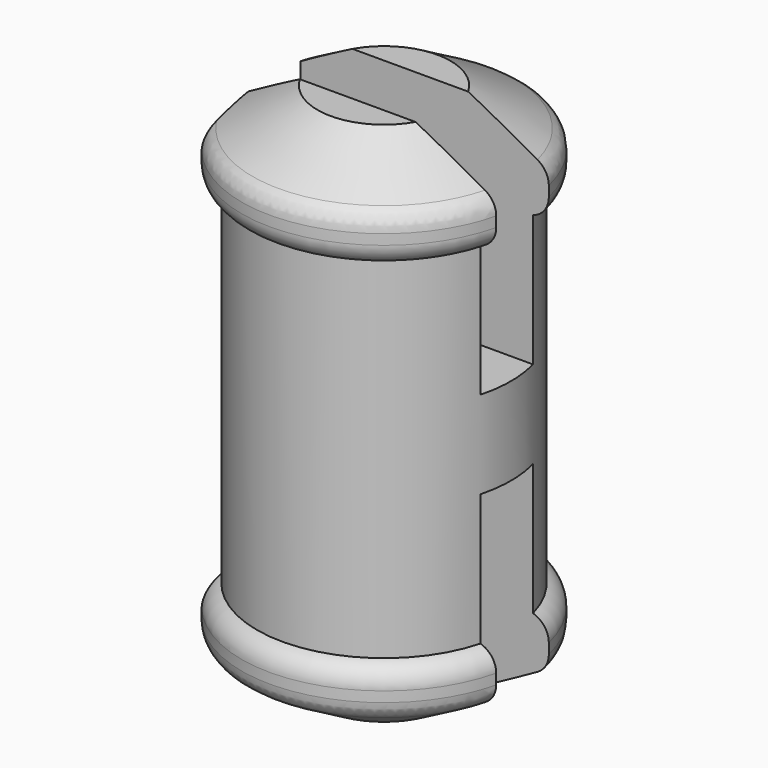
from build123d import *

# Parameters (mm, degrees)
F0_R         = 3.25
F1_DEPTH     = 2
F2_R         = 2.9
F3_DEPTH     = 8
F4_R         = 3.25
F5_DEPTH     = 2
F8_DEPTH     = 5
F10_DEPTH    = 5
F11_C1_SIZE2 = 1
F11_C1_SIZE  = 1.7320508076
F11_C2_SIZE2 = 1
F11_C2_SIZE  = 1.7320508076
F12_C1_SIZE2 = 1
F12_C1_SIZE  = 1.7320508076
F12_C2_SIZE2 = 1
F12_C2_SIZE  = 1.7320508076
F13_R        = 0.5
F15_DEPTH    = 25


# Not quite as in the source:
# - a fillet or chamfer that OpenCascade refuses, or shapes differently, is made with other operations: its cross-section is extruded or revolved along the edge and cut away or added


with BuildPart() as f1:
    # F0 (on Top) → F1 (new body)
    with BuildSketch(Plane.XY):
        Circle(F0_R)
    extrude(amount=F1_DEPTH)

    # F2 (on face) → F3 (join)
    with BuildSketch(Plane.XY.offset(2)):
        Circle(F2_R)
    extrude(amount=F3_DEPTH)

    # F4 (on face) → F5 (join)
    with BuildSketch(Plane.XY.offset(10)):
        Circle(F4_R)
    extrude(amount=F5_DEPTH)

    # F6: fillet of radius 0.5 on 2 edges, made by hand

    # F6_s1 → F6_t2 (revolve, cut)
    with BuildSketch(Plane.XZ):
        with BuildLine():
            ThreePointArc((2.9, 2), (3.1531128874, 1.8188343884), (3.25, 1.5230303993))
            Line((3.25, 1.5230303993), (3.25, 2))
            Line((3.25, 2), (2.9, 2))
        make_face()
    revolve(axis=Axis((0, 0, 2), (0, 0, 1)), mode=Mode.SUBTRACT)

    # F6_s3 → F6_t4 (revolve, cut)
    with BuildSketch(Plane.XZ):
        with BuildLine():
            ThreePointArc((3.25, 10.4769696007), (3.1531128874, 10.1811656116), (2.9, 10))
            Line((2.9, 10), (3.25, 10))
            Line((3.25, 10), (3.25, 10.4769696007))
        make_face()
    revolve(axis=Axis((0, 0, 10), (0, 0, 1)), mode=Mode.SUBTRACT)

    # F7 (on face) → F8 (cut)
    with BuildSketch(Plane(origin=(0, 0, 0), x_dir=(1, 0, 0), z_dir=(0, 0, -1))):
        with BuildLine():
            ThreePointArc((-3.1622776602, 0.75), (-3.25, 0), (-3.1622776602, -0.75))
            Line((-3.1622776602, -0.75), (3.1622776602, -0.75))
            ThreePointArc((3.1622776602, -0.75), (3.25, 0), (3.1622776602, 0.75))
            Line((3.1622776602, 0.75), (-3.1622776602, 0.75))
        make_face()
    extrude(amount=-F8_DEPTH, mode=Mode.SUBTRACT)

    # F9 (on face) → F10 (cut)
    with BuildSketch(Plane.XY.offset(12)):
        with BuildLine():
            ThreePointArc((-3.1622776602, 0.75), (-3.25, 0), (-3.1622776602, -0.75))
            Line((-3.1622776602, -0.75), (3.1622776602, -0.75))
            ThreePointArc((3.1622776602, -0.75), (3.25, 0), (3.1622776602, 0.75))
            Line((3.1622776602, 0.75), (-3.1622776602, 0.75))
        make_face()
    extrude(amount=-F10_DEPTH, mode=Mode.SUBTRACT)

    # F11: chamfer of 1 x 1.7320508076 on 2 edges, made by hand

    # F11_c1
    f11_c1_edges = [f1.edges().sort_by_distance(p)[0] for p in [
        (0, 3.25, 0),
    ]]
    f11_c1_side = f1.faces().sort_by_distance((0, 3.23, 0))[0]
    chamfer(f11_c1_edges, length=F11_C1_SIZE, length2=F11_C1_SIZE2, reference=f11_c1_side)

    # F11_c2
    f11_c2_edges = [f1.edges().sort_by_distance(p)[0] for p in [
        (0, -3.25, 0),
    ]]
    f11_c2_side = f1.faces().sort_by_distance((0, -3.23, 0))[0]
    chamfer(f11_c2_edges, length=F11_C2_SIZE, length2=F11_C2_SIZE2, reference=f11_c2_side)

    # F12: chamfer of 1 x 1.7320508076 on 2 edges, made by hand

    # F12_c1
    f12_c1_edges = [f1.edges().sort_by_distance(p)[0] for p in [
        (0, -3.25, 12),
    ]]
    f12_c1_side = f1.faces().sort_by_distance((0, -3.23, 12))[0]
    chamfer(f12_c1_edges, length=F12_C1_SIZE, length2=F12_C1_SIZE2, reference=f12_c1_side)

    # F12_c2
    f12_c2_edges = [f1.edges().sort_by_distance(p)[0] for p in [
        (0, 3.25, 12),
    ]]
    f12_c2_side = f1.faces().sort_by_distance((0, 3.23, 12))[0]
    chamfer(f12_c2_edges, length=F12_C2_SIZE, length2=F12_C2_SIZE2, reference=f12_c2_side)

    # F13
    f13_edges = [f1.edges().sort_by_distance(p)[0] for p in [
        (0, -3.25, 11),
        (0, 3.25, 11),
        (0, -3.25, 1),
        (0, 3.25, 1),
    ]]
    fillet(f13_edges, radius=F13_R)

    # F14 (on face) → F15 (cut)
    with BuildSketch(Plane.XY.offset(12)):
        with BuildLine():
            Line((-2.5, -2.0766559657), (-2.5, 2.0766559657))
            ThreePointArc((-2.5, 2.0766559657), (-3.25, 0), (-2.5, -2.0766559657))
        make_face()
    extrude(amount=-F15_DEPTH, mode=Mode.SUBTRACT)


solid = f1.part
